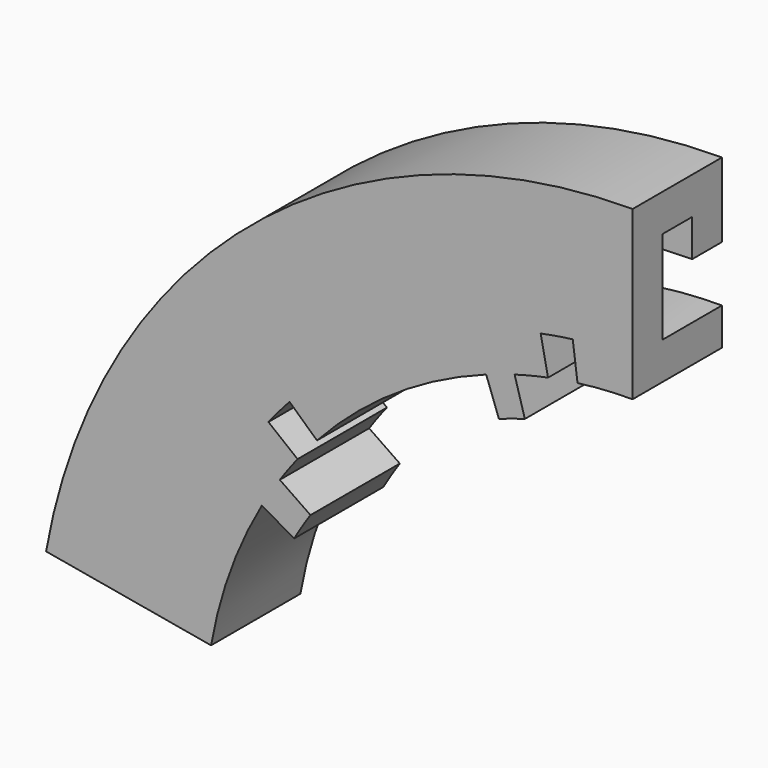
from build123d import *

# Parameters (mm, degrees)
F1_DEPTH = 10
F3_DEPTH = 5
F5_DEPTH = 15
F8_DEPTH = 15
F9_DEPTH = 25


# Not quite as in the source:
# - a feature names something its author has since deleted; it is built from what else it names


with BuildPart() as f1:
    # F0 (on Front) → F1 (new body, symmetric)
    with BuildSketch(Plane.XZ):
        with BuildLine():
            Line((-62.5, -30), (-62.5, 0))
            Line((-62.5, 0), (-75, 0))
            ThreePointArc((-75, 0), (-73.4179734698, -15.3232232767), (-68.7386354243, -30))
            Line((-68.7386354243, -30), (-62.5, -30))
        make_face()
        with BuildLine():
            ThreePointArc((-68.7386354243, -30), (-73.4179734698, -15.3232232767), (-75, 0))
            Line((-75, 0), (-75, -30))
            Line((-75, -30), (-68.7386354243, -30))
        make_face()
        with BuildLine():
            Line((-75, 0), (-62.5, 0))
            ThreePointArc((-62.5, 0), (-44.1941738242, 44.1941738242), (0, 62.5))
            Line((0, 62.5), (0, 75))
            ThreePointArc((0, 75), (-53.033008589, 53.033008589), (-75, 0))
        make_face()
        with BuildLine():
            ThreePointArc((0, 62.5), (23.9177145228, 57.742470782), (44.1941738242, 44.1941738242))
            Line((44.1941738242, 44.1941738242), (44.1941738242, 56.6941738242))
            Line((44.1941738242, 56.6941738242), (49.0995993303, 56.6941738242))
            ThreePointArc((49.0995993303, 56.6941738242), (26.2005435362, 70.274686185), (0, 75))
            Line((0, 75), (0, 62.5))
        make_face()
        with BuildLine():
            Line((44.1941738242, 56.6941738242), (44.1941738242, 44.1941738242))
            Line((44.1941738242, 44.1941738242), (53.033008589, 53.033008589))
            ThreePointArc((53.033008589, 53.033008589), (51.0991040315, 54.8988302897), (49.0995993303, 56.6941738242))
            Line((49.0995993303, 56.6941738242), (44.1941738242, 56.6941738242))
        make_face()
        with BuildLine():
            ThreePointArc((49.0995993303, 56.6941738242), (51.0991040315, 54.8988302897), (53.033008589, 53.033008589))
            ThreePointArc((53.033008589, 53.033008589), (56.9861303035, 48.7604445533), (60.5959982177, 44.1941738242))
            Line((60.5959982177, 44.1941738242), (79.1941738242, 44.1941738242))
            Line((79.1941738242, 44.1941738242), (79.1941738242, 56.6941738242))
            Line((79.1941738242, 56.6941738242), (49.0995993303, 56.6941738242))
        make_face()
        with BuildLine():
            Line((53.033008589, 53.033008589), (44.1941738242, 44.1941738242))
            Line((44.1941738242, 44.1941738242), (60.5959982177, 44.1941738242))
            ThreePointArc((60.5959982177, 44.1941738242), (56.9861303035, 48.7604445533), (53.033008589, 53.033008589))
        make_face()
    extrude(amount=F1_DEPTH, both=True)

    # F2 (on Front) → F3 (cut, symmetric)
    with BuildSketch(Plane.XZ):
        with BuildLine():
            Line((45.9241320293, 52.8296706156), (49.2044271743, 56.6032185167))
            ThreePointArc((49.2044271743, 56.6032185167), (-31.1019931992, 68.2470953157), (-75, 0))
            Line((-75, 0), (-70, 0))
            ThreePointArc((-70, 0), (-29.0285269859, 63.6972889614), (45.9241320293, 52.8296706156))
        make_face()
    extrude(amount=F3_DEPTH, both=True, mode=Mode.SUBTRACT)


with BuildPart() as f5:
    # F4 (on Front) → F5 (new body)
    with BuildSketch(Plane.XZ):
        with BuildLine():
            ThreePointArc((-56.6264457982, 9.9847702158), (-36.960287557, 44.0475554793), (0, 57.5))
            Line((0, 57.5), (0, 80))
            ThreePointArc((0, 80), (-51.4230087749, 61.2835554495), (-78.784620241, 13.8918542134))
            Line((-78.784620241, 13.8918542134), (-56.6264457982, 9.9847702158))
        make_face()
    extrude(amount=F5_DEPTH)

    # F6: cut F1
    add(f1.part, mode=Mode.SUBTRACT)

    # F7 (on face) → F8 (join, through all)
    with BuildSketch(Plane.XZ.offset(15)):
        with BuildLine():
            ThreePointArc((-47.389204942, 32.5655224887), (-48.6302678935, 30.6813794443), (-49.7964607176, 28.75))
            Line((-49.7964607176, 28.75), (-45.4663336987, 26.25))
            ThreePointArc((-45.4663336987, 26.25), (-44.4015489462, 28.0134334057), (-43.2684045123, 29.7337379245))
            Line((-43.2684045123, 29.7337379245), (-47.389204942, 32.5655224887))
        make_face()
        with BuildLine():
            Line((-14.4709611804, 50.4662390368), (-15.8491479595, 55.2725475165))
            ThreePointArc((-15.8491479595, 55.2725475165), (-17.7684771766, 54.685749687), (-19.6661582412, 54.0323256952))
            Line((-19.6661582412, 54.0323256952), (-17.9560575246, 49.3338625913))
            ThreePointArc((-17.9560575246, 49.3338625913), (-16.2233922047, 49.9304671055), (-14.4709611804, 50.4662390368))
        make_face()
    extrude(amount=-F8_DEPTH)

    # F7 (on face) → F9 (cut)
    with BuildSketch(Plane.XZ.offset(15)):
        with BuildLine():
            Line((-48.9153382675, 38.9042373293), (-45.0021112061, 35.7918983429))
            ThreePointArc((-45.0021112061, 35.7918983429), (-43.7255778977, 37.3406459172), (-42.395771708, 38.8438996663))
            Line((-42.395771708, 38.8438996663), (-46.0823605522, 42.221630072))
            ThreePointArc((-46.0823605522, 42.221630072), (-47.5278020627, 40.5876586056), (-48.9153382675, 38.9042373293))
        make_face()
        with BuildLine():
            ThreePointArc((-11.3558821654, 56.3674901006), (-9.3817674339, 56.7294671209), (-7.396222464, 57.0223280239))
            Line((-7.396222464, 57.0223280239), (-8.0393722435, 61.9807913303))
            ThreePointArc((-8.0393722435, 61.9807913303), (-10.1975732978, 61.6624642618), (-12.3433501798, 61.269010979))
            Line((-12.3433501798, 61.269010979), (-11.3558821654, 56.3674901006))
        make_face()
    extrude(amount=-F9_DEPTH, mode=Mode.SUBTRACT)


solid = f5.part
